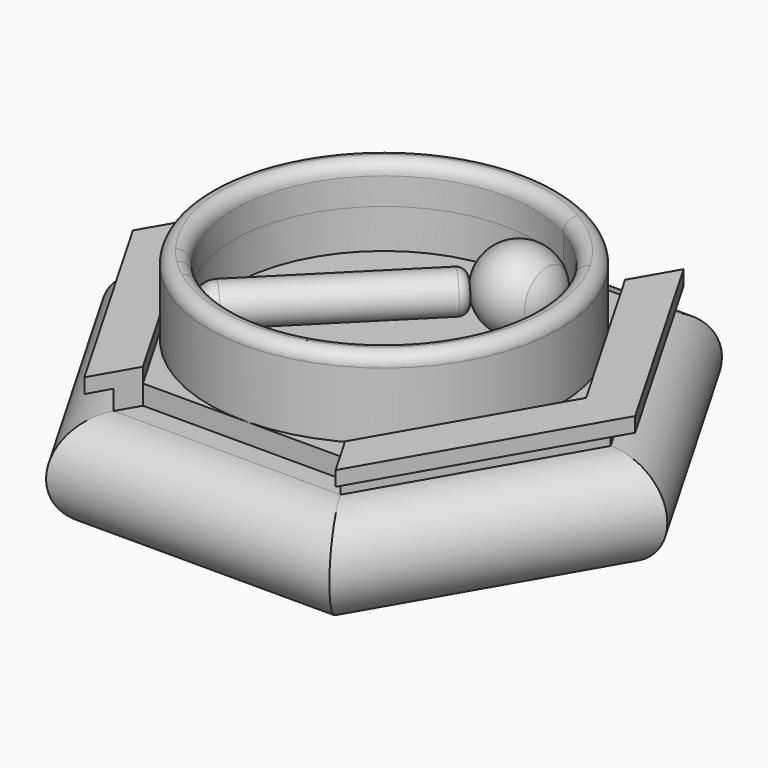
from build123d import *

# Parameters (mm, degrees)
F1_DEPTH  = 12.7
F3_DEPTH  = 25.4
F6_DEPTH  = 25.4
F9_DEPTH  = 25.4
F11_DEPTH = 1.778
F12_DEPTH = 1.016
F13_DEPTH = 1.016
F18_R     = 1.015
F19_R     = 0.508
F15_R     = 9.0601477372
F20_DEPTH = 2.032
F21_R     = 0.635
F22_R     = 0.63499


# Not quite as in the source:
# - a fillet or chamfer is up to 0.001 mm smaller than in the source, because OpenCascade refuses the exact size


with BuildPart() as f1:
    # F0 (on Front) → F1 (new body, symmetric)
    with BuildSketch(Plane.XZ):
        with BuildLine():
            Line((-12.7, 0), (0, 0))
            Line((0, 0), (12.7, 0))
            ThreePointArc((12.7, 0), (15.24, 2.54), (12.7, 5.08))
            Line((12.7, 5.08), (-12.7, 5.08))
            ThreePointArc((-12.7, 5.08), (-15.24, 2.54), (-12.7, 0))
        make_face()
    extrude(amount=F1_DEPTH, both=True)

    # F2 (on Right) → F3 (cut, symmetric)
    with BuildSketch(Plane.YZ):
        with BuildLine():
            ThreePointArc((10.16, 5.08), (12.7, 2.54), (10.16, 0))
            Line((10.16, 0), (29.21, 0))
            Line((29.21, 0), (29.21, 5.08))
            Line((29.21, 5.08), (10.16, 5.08))
        make_face()
        with BuildLine():
            ThreePointArc((-10.16, 0), (-12.7, 2.54), (-10.16, 5.08))
            Line((-10.16, 5.08), (-29.21, 5.08))
            Line((-29.21, 5.08), (-29.21, 0))
            Line((-29.21, 0), (-10.16, 0))
        make_face()
    extrude(amount=F3_DEPTH, both=True, mode=Mode.SUBTRACT)

    # F5 (on line) → F6 (cut, symmetric)
    with BuildSketch(Plane(origin=(0, 0, 0), x_dir=(-0.8660254038, -0.5, 0), z_dir=(-0.5, 0.8660254038, 0))):
        with BuildLine():
            ThreePointArc((10.16, 5.08), (12.7, 2.54), (10.16, 0))
            Line((10.16, 0), (29.21, 0))
            Line((29.21, 0), (29.21, 5.08))
            Line((29.21, 5.08), (10.16, 5.08))
        make_face()
        with BuildLine():
            ThreePointArc((-10.16, 0), (-12.7, 2.54), (-10.16, 5.08))
            Line((-10.16, 5.08), (-29.21, 5.08))
            Line((-29.21, 5.08), (-29.21, 0))
            Line((-29.21, 0), (-10.16, 0))
        make_face()
    extrude(amount=F6_DEPTH, both=True, mode=Mode.SUBTRACT)

    # F8 (on line) → F9 (cut, symmetric)
    with BuildSketch(Plane(origin=(0, 0, 0), x_dir=(-0.8660254038, 0.5, 0), z_dir=(0.5, 0.8660254038, 0))):
        with BuildLine():
            ThreePointArc((10.16, 5.08), (12.7, 2.54), (10.16, 0))
            Line((10.16, 0), (29.21, 0))
            Line((29.21, 0), (29.21, 5.08))
            Line((29.21, 5.08), (10.16, 5.08))
        make_face()
        with BuildLine():
            ThreePointArc((-10.16, 0), (-12.7, 2.54), (-10.16, 5.08))
            Line((-10.16, 5.08), (-29.21, 5.08))
            Line((-29.21, 5.08), (-29.21, 0))
            Line((-29.21, 0), (-10.16, 0))
        make_face()
    extrude(amount=F9_DEPTH, both=True, mode=Mode.SUBTRACT)

    # F10 (on face) → F11 (join)
    with BuildSketch(Plane.XY.offset(5.08)):
        Polygon((-5.230878735, 9.0601477372), (-5.865878735, 10.16), (-11.7317574699, 0), (-5.865878735, -10.16), (-5.230878735, -9.0601477372), (-10.4617574699, 0), align=None)
        Polygon((-11.7317574699, 0), (-5.865878735, 10.16), (-6.500878735, 11.2598522628), (-13.0017574699, 0), (-6.500878735, -11.2598522628), (-5.865878735, -10.16), align=None)
        Polygon((11.7317574699, 0), (5.865878735, 10.16), (5.230878735, 9.0601477372), (10.4617574699, 0), (5.230878735, -9.0601477372), (5.865878735, -10.16), align=None)
        Polygon((6.500878735, 11.2598522628), (5.865878735, 10.16), (11.7317574699, 0), (5.865878735, -10.16), (6.500878735, -11.2598522628), (13.0017574699, 0), align=None)
    extrude(amount=F11_DEPTH)

    # F10 (on face) → F12 (cut)
    with BuildSketch(Plane.XY.offset(5.08)):
        Polygon((6.500878735, 11.2598522628), (5.865878735, 10.16), (11.7317574699, 0), (5.865878735, -10.16), (6.500878735, -11.2598522628), (13.0017574699, 0), align=None)
        Polygon((-11.7317574699, 0), (-5.865878735, 10.16), (-6.500878735, 11.2598522628), (-13.0017574699, 0), (-6.500878735, -11.2598522628), (-5.865878735, -10.16), align=None)
    extrude(amount=F12_DEPTH, mode=Mode.SUBTRACT)

    # F10 (on face) → F13 (join)
    with BuildSketch(Plane.XY.offset(5.08)):
        Polygon((10.4617574699, 0), (5.230878735, 9.0601477372), (-5.230878735, 9.0601477372), (-10.4617574699, 0), (-5.230878735, -9.0601477372), (5.230878735, -9.0601477372), align=None)
    extrude(amount=F13_DEPTH)


with BuildPart() as f16:
    # F15 (on offset) → F16 (revolve)
    with BuildSketch(Plane.XY.offset(8.128)):
        with BuildLine():
            ThreePointArc((5.9129300653, 3.8809300653), (5.7582532754, 4.6585427999), (5.3177710447, 5.3177710447))
            ThreePointArc((5.3177710447, 5.3177710447), (3.8809300653, 5.9129300653), (2.4440890859, 5.3177710447))
            ThreePointArc((2.4440890859, 5.3177710447), (2.0036068552, 4.6585427999), (1.8489300653, 3.8809300653))
            Line((1.8489300653, 3.8809300653), (5.9129300653, 3.8809300653))
        make_face()
    revolve(axis=Axis((3.8809300653, 3.8809300653, 8.128), (1, 0, 0)))


with BuildPart() as f17:
    # F15 (on offset) → F17 (revolve)
    with BuildSketch(Plane.XY.offset(8.128)):
        with BuildLine():
            ThreePointArc((-6.1798372366, -4.7429962572), (-5.8566710625, -5.1367115778), (-5.5084662914, -5.5084662914))
            Line((-5.5084662914, -5.5084662914), (0, 0))
            Line((0, 0), (2.4440890859, 2.4440890859))
            Line((2.4440890859, 2.4440890859), (1.7256685963, 3.1625095756))
            Line((1.7256685963, 3.1625095756), (-6.1798372366, -4.7429962572))
        make_face()
    revolve(axis=Axis((-2.7542331457, -2.7542331457, 8.128), (-0.7071067812, -0.7071067812, 0)))

    # F18 (radius 1.016 in the source; OpenCascade refuses exactly that, so slightly less here)
    f18_edges = [f17.edges().sort_by_distance(p)[0] for p in [
        (-4.742996, -6.179837, 8.128),
    ]]
    fillet(f18_edges, radius=F18_R)

    # F19
    f19_edges = [f17.edges().sort_by_distance(p)[0] for p in [
        (3.16251, 1.725669, 8.128),
    ]]
    fillet(f19_edges, radius=F19_R)


with BuildPart() as f20:
    # F15 (on offset) → F20 (new body, symmetric)
    with BuildSketch(Plane.XY.offset(8.128)):
        Circle(F15_R)
        with BuildLine():
            ThreePointArc((6.7546120241, 3.8809300653), (7.5268129823, 2.0083545743), (7.7901477372, 0))
            ThreePointArc((7.7901477372, 0), (3.4821359873, -6.9685816874), (-4.6771718494, -6.2298045923))
            ThreePointArc((-4.6771718494, -6.2298045923), (-5.10557424, -5.8838349269), (-5.5084662914, -5.5084662914))
            ThreePointArc((-5.5084662914, -5.5084662914), (-5.8566710625, -5.1367115778), (-6.1798372366, -4.7429962572))
            ThreePointArc((-6.1798372366, -4.7429962572), (-5.8625926511, 5.129952161), (3.8809300653, 6.7546120241))
            ThreePointArc((3.8809300653, 6.7546120241), (5.5084662914, 5.5084662914), (6.7546120241, 3.8809300653))
        make_face(mode=Mode.SUBTRACT)
    extrude(amount=F20_DEPTH, both=True)

    # F21
    f21_edges = [f20.edges().sort_by_distance(p)[0] for p in [
        (-9.060148, 0, 10.16),
    ]]
    fillet(f21_edges, radius=F21_R)

    # F22 (radius 0.635 in the source; OpenCascade refuses exactly that, so slightly less here)
    f22_edges = [f20.edges().sort_by_distance(p)[0] for p in [
        (-5.862593, 5.129952, 10.16),
    ]]
    fillet(f22_edges, radius=F22_R)


solid = Compound([f1.part, f16.part, f17.part, f20.part])
